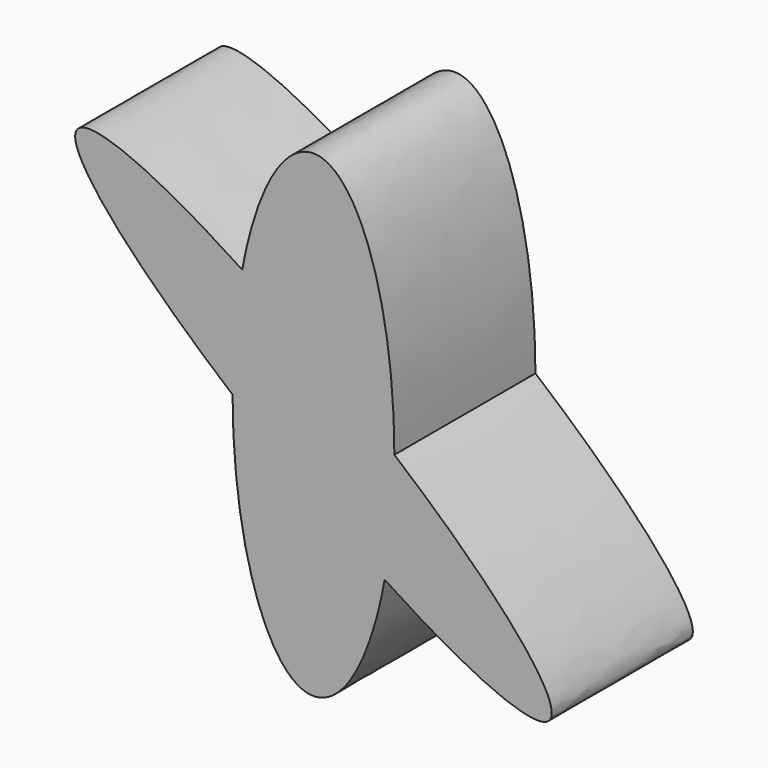
from build123d import *

# Parameters (mm, degrees)
F1_DEPTH = 25.4


with BuildPart() as f1:
    # F0 (on Front) → F1 (new body)
    with BuildSketch(Plane.XZ):
        with BuildLine():
            add(Edge.make_bspline(
                [(-23.7685478879, 10.0557711837), (-2.8513099786, -3.6790146109), (0, 0)],
                knots=[5.1464295715, 5.1464295715, 5.1464295715, 6.2831853072, 6.2831853072, 6.2831853072], degree=2, weights=[1, 0.8427752216, 1]))
            add(Edge.make_bspline(
                [(0, 0), (3.5909872709, 4.6334122688), (-22.3747425204, 26.3469081794)],
                knots=[0, 0, 0, 1.3547963993, 1.3547963993, 1.3547963993], degree=2, weights=[1, 0.779206079, 1]))
            add(Edge.make_bspline(
                [(-23.7685478879, 10.0557711837), (-22.3769478232, 17.6832466322), (-22.3747425204, 26.3469081794)],
                knots=[4.2182941759, 4.2182941759, 4.2182941759, 4.7116374486, 4.7116374486, 4.7116374486], degree=2, weights=[1, 0.9697305037, 1]))
        make_face()
        with BuildLine():
            add(Edge.make_bspline(
                [(-23.7685478879, 10.0557711837), (-22.3769478232, 17.6832466322), (-22.3747425204, 26.3469081794)],
                knots=[4.2182941759, 4.2182941759, 4.2182941759, 4.7116374486, 4.7116374486, 4.7116374486], degree=2, weights=[1, 0.9697305037, 1]))
            add(Edge.make_bspline(
                [(-22.3747425204, 26.3469081794), (-33.252461311, 35.4432557258), (-44.2884452986, 42.6897610607)],
                knots=[1.3547963993, 1.3547963993, 1.3547963993, 2.0048369179, 2.0048369179, 2.0048369179], degree=2, weights=[1, 0.9476442572, 1]))
            add(Edge.make_bspline(
                [(-44.2884452986, 42.6897610607), (-45.6800453633, 35.0622856122), (-45.6822506661, 26.398624065)],
                knots=[1.0767015223, 1.0767015223, 1.0767015223, 1.570044795, 1.570044795, 1.570044795], degree=2, weights=[1, 0.9697305037, 1]))
            add(Edge.make_bspline(
                [(-45.6822506661, 26.398624065), (-34.8045318754, 17.3022765186), (-23.7685478879, 10.0557711837)],
                knots=[4.4963890529, 4.4963890529, 4.4963890529, 5.1464295715, 5.1464295715, 5.1464295715], degree=2, weights=[1, 0.9476442572, 1]))
        make_face()
        with BuildLine():
            add(Edge.make_bspline(
                [(-22.3747425204, 26.3469081794), (-33.252461311, 35.4432557258), (-44.2884452986, 42.6897610607)],
                knots=[1.3547963993, 1.3547963993, 1.3547963993, 2.0048369179, 2.0048369179, 2.0048369179], degree=2, weights=[1, 0.9476442572, 1]))
            add(Edge.make_bspline(
                [(-22.3747425204, 26.3469081794), (-22.3659777675, 60.7797540724), (-34.0284965932, 60.7797540724)],
                knots=[4.7116374486, 4.7116374486, 4.7116374486, 6.2831853072, 6.2831853072, 6.2831853072], degree=2, weights=[1, 0.7068410247, 1]))
            add(Edge.make_bspline(
                [(-34.0284965932, 60.7797540724), (-40.9880039381, 60.7797540724), (-44.2884452986, 42.6897610607)],
                knots=[0, 0, 0, 1.0767015223, 1.0767015223, 1.0767015223], degree=2, weights=[1, 0.8585554476, 1]))
        make_face()
        with BuildLine():
            add(Edge.make_bspline(
                [(-45.6822506661, 26.398624065), (-45.689076912, -0.4186836893), (-36.8825765449, -6.9864162792), (-28.0760761777, -13.554148869), (-23.7685478879, 10.0557711837)],
                knots=[1.570044795, 1.570044795, 1.570044795, 2.8941694854, 2.8941694854, 4.2182941759, 4.2182941759, 4.2182941759], degree=2, weights=[1, 0.7887260938, 1, 0.7887260938, 1]))
            add(Edge.make_bspline(
                [(-45.6822506661, 26.398624065), (-34.8045318754, 17.3022765186), (-23.7685478879, 10.0557711837)],
                knots=[4.4963890529, 4.4963890529, 4.4963890529, 5.1464295715, 5.1464295715, 5.1464295715], degree=2, weights=[1, 0.9476442572, 1]))
        make_face()
        with BuildLine():
            add(Edge.make_bspline(
                [(-44.2884452986, 42.6897610607), (-45.6800453633, 35.0622856122), (-45.6822506661, 26.398624065)],
                knots=[1.0767015223, 1.0767015223, 1.0767015223, 1.570044795, 1.570044795, 1.570044795], degree=2, weights=[1, 0.9697305037, 1]))
            add(Edge.make_bspline(
                [(-44.2884452986, 42.6897610607), (-141.479830545, 106.5080750863), (-45.6822506661, 26.398624065)],
                knots=[2.0048369179, 2.0048369179, 2.0048369179, 4.4963890529, 4.4963890529, 4.4963890529], degree=2, weights=[1, 0.3193279845, 1]))
        make_face()
    extrude(amount=F1_DEPTH)


solid = f1.part
